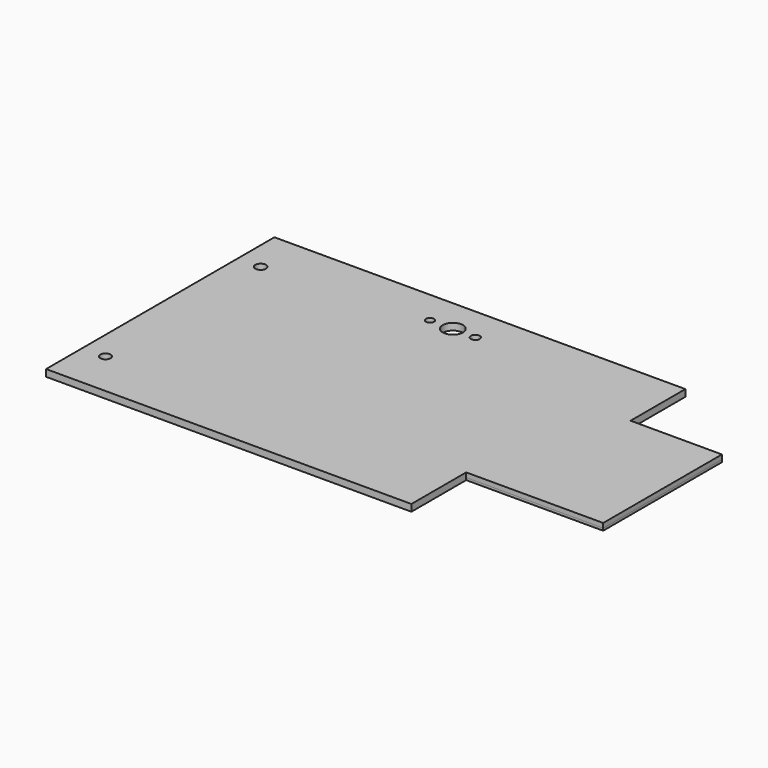
from build123d import *

# Parameters (mm, degrees)
F0_W     = 180
F0_H     = 30
F0_R     = 2.3391107882
F0_R_2   = 1.7779977582
F0_R_3   = 4.4113535935
F0_R_4   = 1.9309092274
F0_W_2   = 160
F0_R_5   = 2.2327370736
F1_DEPTH = 3
F2_DEPTH = 1


# Not quite as in the source:
# - a feature names something its author has since deleted; it is built from what else it names


with BuildPart() as f1:
    # F0 (on Top) → F1 (new body)
    with BuildSketch(Plane.XY):
        with Locations((-0.42535007, 48.7836791575)):
            Rectangle(F0_W, F0_H)
        with Locations((-80.42535007, 43.7836791575)):
            Circle(F0_R, mode=Mode.SUBTRACT)
        with Locations((-10.42535007, 48.9865408171)):
            Circle(F0_R_2, mode=Mode.SUBTRACT)
        with Locations((-0.42535007, 48.9865408171)):
            Circle(F0_R_3, mode=Mode.SUBTRACT)
        with Locations((9.57464993, 48.7836791575)):
            Circle(F0_R_4, mode=Mode.SUBTRACT)
        Polygon((89.57464993, 33.7836791575), (-90.42535007, 33.7836791575), (-90.42535007, -31.2163208425), (69.57464993, -31.2163208425), (129.57464993, -31.2163208425), (129.57464993, 33.7836791575), align=None)
        with Locations((-10.42535007, -46.2163208425)):
            Rectangle(F0_W_2, F0_H)
        with Locations((-80.42535007, -41.2163208425)):
            Circle(F0_R_5, mode=Mode.SUBTRACT)
    extrude(amount=F1_DEPTH)


with BuildPart() as f2:
    # F0 (on Top) → F2 (new body)
    with BuildSketch(Plane.XY):
        Polygon((89.57464993, 33.7836791575), (-90.42535007, 33.7836791575), (-90.42535007, -31.2163208425), (69.57464993, -31.2163208425), (129.57464993, -31.2163208425), (129.57464993, 33.7836791575), align=None)
    extrude(amount=F2_DEPTH)


solid = Compound([f1.part, f2.part])
